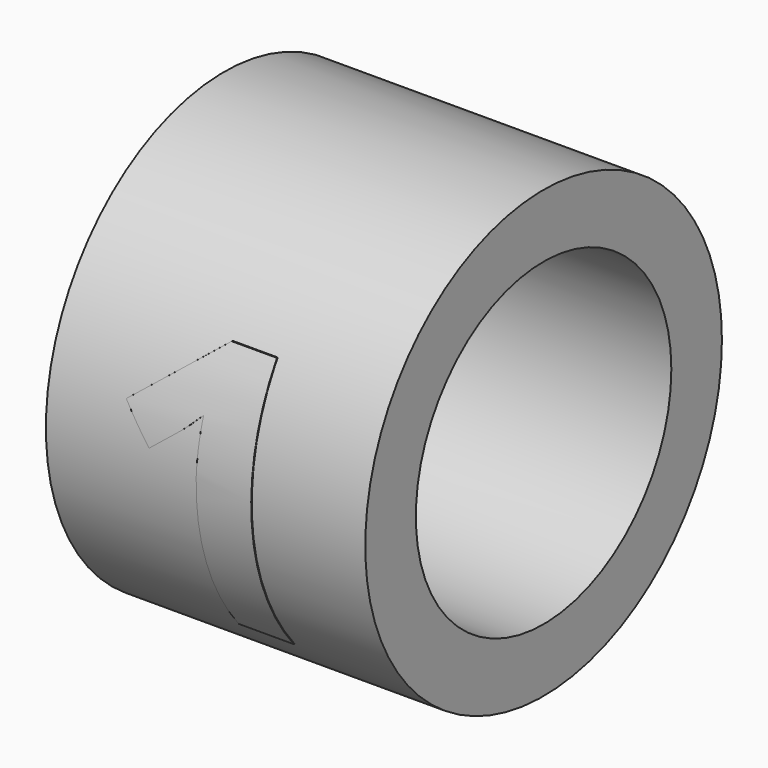
from build123d import *

# Parameters (mm, degrees)
F0_R         = 1.75
F0_R_2       = 1.745
F0_R_3       = 1.25
F1_DEPTH     = 2.5
F2_TEXT_SIZE = 2.8570699214
F3_REACH     = 4.0277504888
F4_DEPTH     = 2.5


# Not quite as in the source:
# - Text() gives the source's letters only with a copy of the font that has no kerning and outlines rounded to 1/6400 em; it was checked with that copy


with BuildPart() as f1:
    # F0 (on Right) → F1 (new body)
    with BuildSketch(Plane.YZ):
        Circle(F0_R)
        Circle(F0_R_2, mode=Mode.SUBTRACT)
        Circle(F0_R_2)
        Circle(F0_R_3, mode=Mode.SUBTRACT)
    extrude(amount=F1_DEPTH)

    f3_end = f1.faces().sort_by_distance((1.25, -1.75, 0))[0]
    # F2 (on Front) → F3 (intersect, up to a face of the model that its end follows)
    with BuildSketch(Plane.XZ):
        with Locations((0.4309935612, -1.1343103251)):
            Text('1', F2_TEXT_SIZE, font='Open Sans', font_style=FontStyle.BOLD, text_align=(TextAlign.LEFT, TextAlign.BOTTOM))
    f3_long = extrude(amount=F3_REACH, mode=Mode.PRIVATE)
    add(split(f3_long, bisect_by=f3_end, keep=Keep.BOTTOM, mode=Mode.PRIVATE), mode=Mode.INTERSECT)


with BuildPart() as f4:
    # F0 (on Right) → F4 (new body)
    with BuildSketch(Plane.YZ):
        Circle(F0_R_2)
        Circle(F0_R_3, mode=Mode.SUBTRACT)
    extrude(amount=F4_DEPTH)


solid = Compound([f1.part, f4.part])
